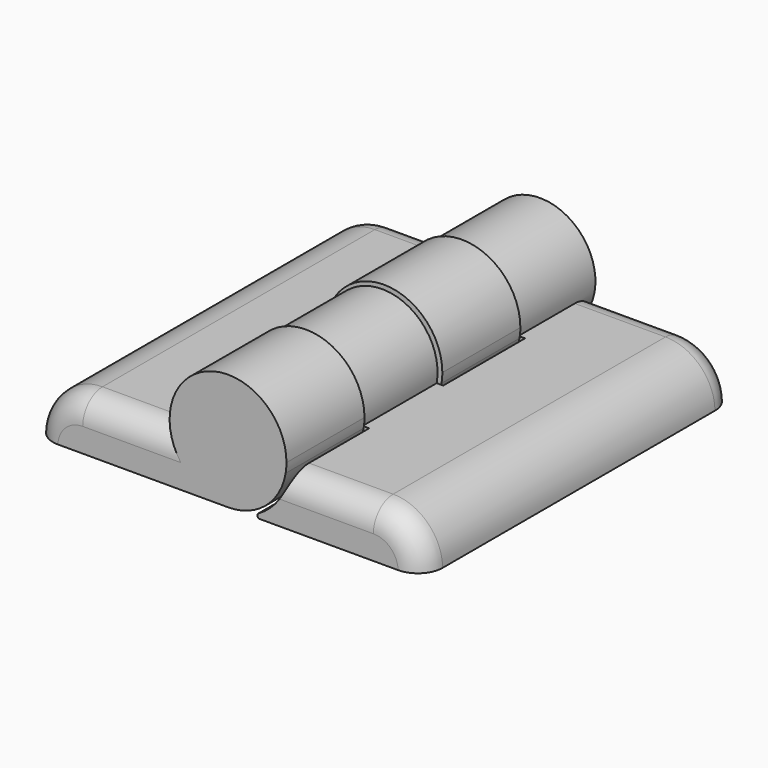
from build123d import *

# Parameters (mm, degrees)
F3_DEPTH     = 10.0076
F4_DEPTH     = 40.005
F6_START     = -19.9898
F6_DEPTH     = 10.0076
F7_DEPTH     = 10.0076
F9_START     = 20.2438
F2_R         = 3.2004
F9_DEPTH     = 9.4996
F10_DEPTH    = 10.2616
F11_START    = 20.0152
F11_DEPTH    = 9.9822
F12_START    = -19.7612
F12_DEPTH    = 11.6078
F13_DEPTH    = 9.7536
F14_T1_DEPTH = 13.1863686745
F15_T1_DEPTH = 65.405
F16_R        = 2.54


# Not quite as in the source:
# - a fillet or chamfer that OpenCascade refuses, or shapes differently, is made with other operations: its cross-section is extruded or revolved along the edge and cut away or added


with BuildPart() as f3:
    # F0 (on Front) → F3 (new body)
    with BuildSketch(Plane.XZ):
        with BuildLine():
            ThreePointArc((-5.9119830007, 5.0038), (-3.8726462994, 1.4188735822), (0, 0))
            ThreePointArc((0, 0), (3.8726462994, 1.4188735822), (5.9119830007, 5.0038))
            ThreePointArc((5.9119830007, 5.0038), (5.9737602169, 5.4973887019), (5.9944, 5.9944))
            ThreePointArc((5.9944, 5.9944), (-0.4970112981, 11.9681602169), (-5.9119830007, 5.0038))
        make_face()
        with BuildLine():
            ThreePointArc((-0.3048, 3.0127385839), (0, 8.9916), (0.3048, 3.0127385839))
            Line((0.3048, 3.0127385839), (0.3048, 2.808547348))
            ThreePointArc((0.3048, 2.808547348), (0, 2.794), (-0.3048, 2.808547348))
            Line((-0.3048, 2.808547348), (-0.3048, 3.0127385839))
        make_face(mode=Mode.SUBTRACT)
        with BuildLine():
            Line((-19.9898, 0), (0, 0))
            ThreePointArc((0, 0), (-3.8726462994, 1.4188735822), (-5.9119830007, 5.0038))
            Line((-5.9119830007, 5.0038), (-19.9898, 5.0038))
            Line((-19.9898, 5.0038), (-19.9898, 0))
        make_face()
    extrude(amount=-F3_DEPTH)

    # F0 (on Front) → F4 (join)
    with BuildSketch(Plane.XZ):
        with BuildLine():
            Line((0.3048, 2.808547348), (0.3048, 3.0127385839))
            ThreePointArc((0.3048, 3.0127385839), (0, 8.9916), (-0.3048, 3.0127385839))
            Line((-0.3048, 3.0127385839), (-0.3048, 2.808547348))
            ThreePointArc((-0.3048, 2.808547348), (0, 2.794), (0.3048, 2.808547348))
        make_face()
    extrude(amount=-F4_DEPTH)

    # F0 (on Front) → F6 (join)
    with BuildSketch(Plane.XZ.offset(F6_START)):
        with BuildLine():
            ThreePointArc((-5.9119830007, 5.0038), (-3.8726462994, 1.4188735822), (0, 0))
            ThreePointArc((0, 0), (3.8726462994, 1.4188735822), (5.9119830007, 5.0038))
            ThreePointArc((5.9119830007, 5.0038), (5.9737602169, 5.4973887019), (5.9944, 5.9944))
            ThreePointArc((5.9944, 5.9944), (-0.4970112981, 11.9681602169), (-5.9119830007, 5.0038))
        make_face()
        with BuildLine():
            ThreePointArc((-0.3048, 3.0127385839), (0, 8.9916), (0.3048, 3.0127385839))
            Line((0.3048, 3.0127385839), (0.3048, 2.808547348))
            ThreePointArc((0.3048, 2.808547348), (0, 2.794), (-0.3048, 2.808547348))
            Line((-0.3048, 2.808547348), (-0.3048, 3.0127385839))
        make_face(mode=Mode.SUBTRACT)
        with BuildLine():
            Line((-19.9898, 0), (0, 0))
            ThreePointArc((0, 0), (-3.8726462994, 1.4188735822), (-5.9119830007, 5.0038))
            Line((-5.9119830007, 5.0038), (-19.9898, 5.0038))
            Line((-19.9898, 5.0038), (-19.9898, 0))
        make_face()
    extrude(amount=-F6_DEPTH)

    # F2 (on offset) → F7 (join)
    with BuildSketch(Plane.XZ.offset(-40.005)):
        with BuildLine():
            ThreePointArc((-1.5118372742, 0.1937811178), (-4.4229342387, 1.9483545134), (-5.9119830007, 5.0038))
            Line((-5.9119830007, 5.0038), (-19.9898, 5.0038))
            Line((-19.9898, 5.0038), (-19.9898, 0))
            Line((-19.9898, 0), (-1.5366753453, 0))
            ThreePointArc((-1.5366753453, 0), (-1.4389921182, 0.0859617436), (-1.5118372742, 0.1937811178))
        make_face()
    extrude(amount=F7_DEPTH)

    # F2 (on offset) → F9 (join)
    with BuildSketch(Plane.XZ.offset(-40.005).offset(F9_START)):
        with BuildLine():
            Line((0, 0.3048), (0, 0))
            ThreePointArc((0, 0), (3.8726462994, 1.4188735822), (5.9119830007, 5.0038))
            Line((5.9119830007, 5.0038), (5.6027011164, 5.0038))
            ThreePointArc((5.6027011164, 5.0038), (-3.6561886166, 10.353738592), (0, 0.3048))
        make_face()
        with Locations((0, 5.9944)):
            Circle(F2_R, mode=Mode.SUBTRACT)
        with BuildLine():
            ThreePointArc((5.9119830007, 5.0038), (3.8726462994, 1.4188735822), (0, 0))
            Line((0, 0), (19.9898, 0))
            Line((19.9898, 0), (19.9898, 5.0038))
            Line((19.9898, 5.0038), (5.9119830007, 5.0038))
        make_face()
    extrude(amount=F9_DEPTH)

    # F0 (on Front) → F10 (join)
    with BuildSketch(Plane.XZ):
        with BuildLine():
            ThreePointArc((6.2722573002, 5.0038), (4.8747199854, 1.9250505355), (2.0951536077, 0))
            Line((2.0951536077, 0), (19.9898, 0))
            Line((19.9898, 0), (19.9898, 5.0038))
            Line((19.9898, 5.0038), (6.2722573002, 5.0038))
        make_face()
    extrude(amount=-F10_DEPTH)

    # F2 (on offset) → F11 (join)
    with BuildSketch(Plane.XZ.offset(-40.005).offset(F11_START)):
        with BuildLine():
            ThreePointArc((-1.5118372742, 0.1937811178), (-4.4229342387, 1.9483545134), (-5.9119830007, 5.0038))
            Line((-5.9119830007, 5.0038), (-19.9898, 5.0038))
            Line((-19.9898, 5.0038), (-19.9898, 0))
            Line((-19.9898, 0), (-1.5366753453, 0))
            ThreePointArc((-1.5366753453, 0), (-1.4389921182, 0.0859617436), (-1.5118372742, 0.1937811178))
        make_face()
    extrude(amount=F11_DEPTH)

    # F0 (on Front) → F12 (join)
    with BuildSketch(Plane.XZ.offset(F12_START)):
        with BuildLine():
            ThreePointArc((6.2722573002, 5.0038), (4.8747199854, 1.9250505355), (2.0951536077, 0))
            Line((2.0951536077, 0), (19.9898, 0))
            Line((19.9898, 0), (19.9898, 5.0038))
            Line((19.9898, 5.0038), (6.2722573002, 5.0038))
        make_face()
    extrude(amount=-F12_DEPTH)

    # F2 (on offset) → F13 (join)
    with BuildSketch(Plane.XZ.offset(-40.005)):
        with BuildLine():
            ThreePointArc((5.9119830007, 5.0038), (3.8726462994, 1.4188735822), (0, 0))
            Line((0, 0), (19.9898, 0))
            Line((19.9898, 0), (19.9898, 5.0038))
            Line((19.9898, 5.0038), (5.9119830007, 5.0038))
        make_face()
        with BuildLine():
            Line((0, 0.3048), (0, 0))
            ThreePointArc((0, 0), (3.8726462994, 1.4188735822), (5.9119830007, 5.0038))
            Line((5.9119830007, 5.0038), (5.6027011164, 5.0038))
            ThreePointArc((5.6027011164, 5.0038), (-3.6561886166, 10.353738592), (0, 0.3048))
        make_face()
        with Locations((0, 5.9944)):
            Circle(F2_R, mode=Mode.SUBTRACT)
    extrude(amount=F13_DEPTH)

    # F14: fillet of radius 0.254 on 1 edges, made by hand

    # F14_s2 → F14_t1 (cut)
    with BuildSketch(Plane.XZ.offset(-10.2616)):
        with BuildLine():
            ThreePointArc((3.1394818053, 0.4747846154), (3.0195052872, 0.1890511444), (3.2650610775, 0))
            Line((3.2650610775, 0), (2.0951536077, 0))
            ThreePointArc((2.0951536077, 0), (2.628061469, 0.2137605098), (3.1394818053, 0.4747846154))
        make_face()
    extrude(amount=F14_T1_DEPTH, mode=Mode.SUBTRACT)

    # F15: fillet of radius 5.08 on 2 edges, made by hand

    # F15_s2 → F15_t1 (cut)
    with BuildSketch(Plane.XZ.offset(-52.705)):
        with BuildLine():
            ThreePointArc((-14.9098, 5.0038), (-18.5019024484, 3.5159024484), (-19.9898, -0.0762))
            Line((-19.9898, -0.0762), (-19.9898, 5.0038))
            Line((-19.9898, 5.0038), (-14.9098, 5.0038))
        make_face()
        with BuildLine():
            ThreePointArc((19.9898, -0.0762), (18.5019024484, 3.5159024484), (14.9098, 5.0038))
            Line((14.9098, 5.0038), (19.9898, 5.0038))
            Line((19.9898, 5.0038), (19.9898, -0.0762))
        make_face()
    extrude(amount=F15_T1_DEPTH, mode=Mode.SUBTRACT)

    # F16
    f16_edges = [f3.edges().sort_by_distance(p)[0] for p in [
        (10.256251, 40.005, 5.0038),
        (-10.410892, 40.005, 5.0038),
        (-10.410892, 0, 5.0038),
        (10.591029, 0, 5.0038),
        (-18.47486, 0, 3.542743),
        (-18.47486, 40.005, 3.542743),
        (18.47486, 40.005, 3.542743),
        (18.47486, 0, 3.542743),
    ]]
    fillet(f16_edges, radius=F16_R)


solid = f3.part
